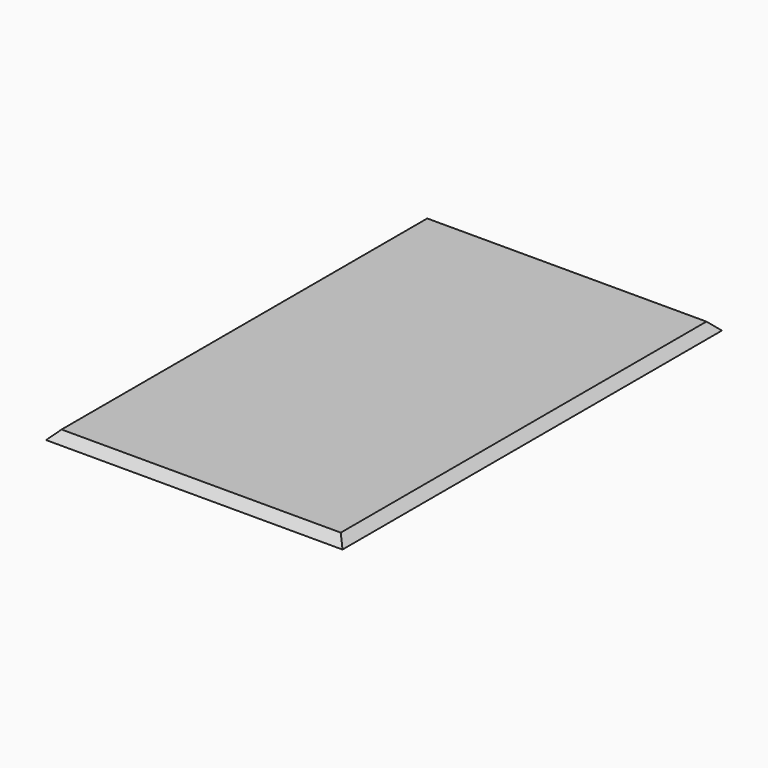
from build123d import *

# Parameters (mm, degrees)
F0_W     = 87.5028249945
F0_H     = 140.0045199912
F1_DEPTH = 2.54
F2_SIZE  = 2.53999


# Not quite as in the source:
# - a fillet or chamfer is up to 0.001 mm smaller than in the source, because OpenCascade refuses the exact size


with BuildPart() as f1:
    # F0 (on Top) → F1 (new body)
    with BuildSketch(Plane.XY):
        Rectangle(F0_W, F0_H)
    extrude(amount=F1_DEPTH)

    # F2 (size 2.54 in the source; OpenCascade refuses exactly that, so slightly less here)
    f2_edges = [f1.edges().sort_by_distance(p)[0] for p in [
        (43.751412, 0, 2.54),
        (-43.751412, 0, 2.54),
        (0, 70.00226, 2.54),
        (0, -70.00226, 2.54),
    ]]
    chamfer(f2_edges, length=F2_SIZE)


solid = f1.part
